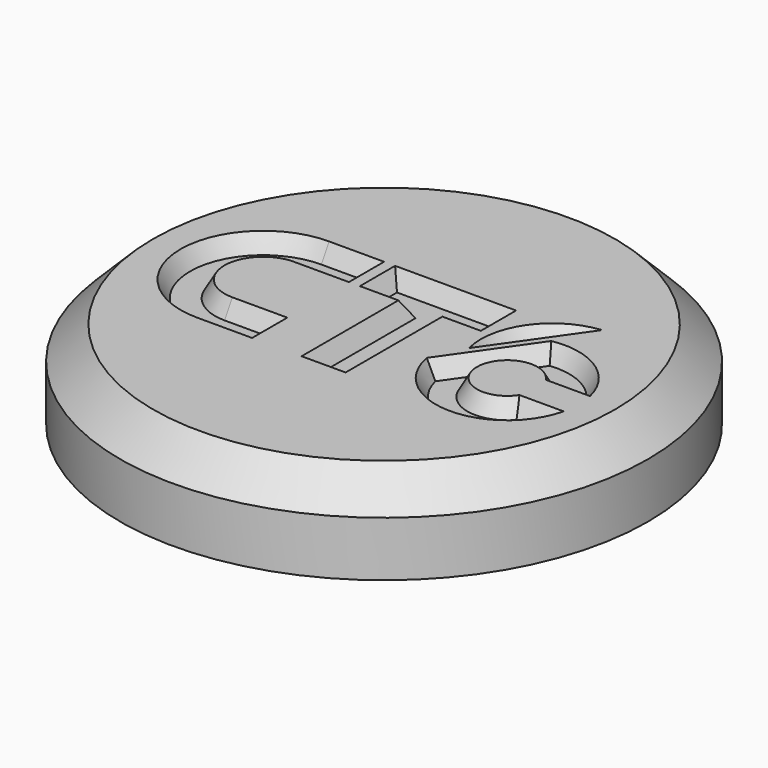
from build123d import *

# Parameters (mm, degrees)
F0_R                     = 24
F1_DEPTH                 = 8
F2_R                     = 21
F3_DEPTH                 = 5.1
F4_SIZE                  = 3
F6_DEPTH                 = 1.5
DRAFT_F6_DRAFTED_ANGLE   = 30
DRAFT_F6_2_DRAFTED_ANGLE = 30
DRAFT_F6_3_DRAFTED_ANGLE = 30
DRAFT_F6_4_DRAFTED_ANGLE = 30


# Not quite as in the source:
# - an extrude with a draft is written as a straight extrude whose walls are then drafted


with BuildPart() as f1:
    # F0 (on Top) → F1 (new body)
    with BuildSketch(Plane.XY):
        Circle(F0_R)
    extrude(amount=F1_DEPTH)

    # F2 (on face) → F3 (cut)
    with BuildSketch(Plane(origin=(0, 0, 0), x_dir=(1, 0, 0), z_dir=(0, 0, -1))):
        Circle(F2_R)
    extrude(amount=-F3_DEPTH, mode=Mode.SUBTRACT)

    # F4
    f4_edges = [f1.edges().sort_by_distance(p)[0] for p in [
        (-24, 0, 8),
    ]]
    chamfer(f4_edges, length=F4_SIZE)


with BuildPart() as f6_drafted:
    # F5 (on face) → F6 (new body)
    with BuildSketch(Plane.XY.offset(8)):
        with BuildLine():
            Line((-6, 7.5), (-11, 7.5))
            ThreePointArc((-11, 7.5), (-18.5, 0), (-11, -7.5))
            Line((-11, -7.5), (-6, -7.5))
            Line((-6, -7.5), (-6, -3.5))
            Line((-6, -3.5), (-11, -3.5))
            ThreePointArc((-11, -3.5), (-14.5, 0), (-11, 3.5))
            Line((-11, 3.5), (-6, 3.5))
            Line((-6, 3.5), (-6, 7.5))
        make_face()
    extrude(amount=-F6_DEPTH)

    # draft_F6_drafted
    draft_f6_drafted_walls = [f6_drafted.faces().sort_by_distance(p)[0] for p in [
        (-8.5, 3.5, 7),
        (-6, 5.5, 7),
        (-8.5, 7.5, 7),
        (-18.5, 0, 7),
        (-8.5, -7.5, 7),
        (-6, -5.5, 7),
        (-8.5, -3.5, 7),
        (-14.5, 0, 7),
    ]]
    draft(draft_f6_drafted_walls, neutral_plane=Plane(origin=(0, 0, 8), x_dir=(1, 0, 0), z_dir=(0, 0, -1)), angle=DRAFT_F6_DRAFTED_ANGLE)


with BuildPart() as f1_1:
    add(f1.part)

    # join_F6_drafted: cut F6_drafted
    add(f6_drafted.part, mode=Mode.SUBTRACT)


with BuildPart() as f6_2_drafted:
    # F5 (on face) → F6, piece 2 (new body)
    with BuildSketch(Plane.XY.offset(8)):
        Polygon((6, 7.5), (0.5, 7.5), (-5, 7.5), (-5, 3.5), (-1.5, 3.5), (-1.5, -7.5), (0.5, -7.5), (2.5, -7.5), (2.5, 3.5), (6, 3.5), align=None)
    extrude(amount=-F6_DEPTH)

    # draft_F6_2_drafted
    draft_f6_2_drafted_walls = [f6_2_drafted.faces().sort_by_distance(p)[0] for p in [
        (0.5, 7.5, 7),
        (4.25, 3.5, 7),
        (2.5, -2, 7),
        (0.5, -7.5, 7),
        (-1.5, -2, 7),
        (-3.25, 3.5, 7),
        (-5, 5.5, 7),
        (6, 5.5, 7),
    ]]
    draft(draft_f6_2_drafted_walls, neutral_plane=Plane(origin=(0, 0, 8), x_dir=(1, 0, 0), z_dir=(0, 0, -1)), angle=DRAFT_F6_2_DRAFTED_ANGLE)


with BuildPart() as f1_2:
    add(f1_1.part)

    # join_F6_2_drafted: cut F6_2_drafted
    add(f6_2_drafted.part, mode=Mode.SUBTRACT)


with BuildPart() as f6_3_drafted:
    # F5 (on face) → F6, piece 3 (new body)
    with BuildSketch(Plane.XY.offset(8)):
        with BuildLine():
            Line((14.3048861143, 0.5), (18.3245553203, 0.5))
            ThreePointArc((18.3245553203, 0.5), (15.575855344, 4.428006868), (10.8818401666, 5.4031022627))
            Line((10.8818401666, 5.4031022627), (5.6006188671, -2.1392634093))
            ThreePointArc((5.6006188671, -2.1392634093), (11.8157923793, -7.4973892874), (18.3245553203, -2.5))
            Line((18.3245553203, -2.5), (14.3048861143, -2.5))
            ThreePointArc((14.3048861143, -2.5), (9.25, -1), (14.3048861143, 0.5))
        make_face()
    extrude(amount=-F6_DEPTH)

    # draft_F6_3_drafted
    draft_f6_3_drafted_walls = [f6_3_drafted.faces().sort_by_distance(p)[0] for p in [
        (16.3147207173, -2.5, 7),
        (9.25, -1, 7),
        (16.3147207173, 0.5, 7),
        (15.575855344, 4.428006868, 7),
        (8.2412295169, 1.6319194267, 7),
        (11.8157923793, -7.4973892874, 7),
    ]]
    draft(draft_f6_3_drafted_walls, neutral_plane=Plane(origin=(0, 0, 8), x_dir=(1, 0, 0), z_dir=(0, 0, -1)), angle=DRAFT_F6_3_DRAFTED_ANGLE)


with BuildPart() as f1_3:
    add(f1_2.part)

    # join_F6_3_drafted: cut F6_3_drafted
    add(f6_3_drafted.part, mode=Mode.SUBTRACT)


with BuildPart() as f6_4_drafted:
    # F5 (on face) → F6, piece 4 (new body)
    with BuildSketch(Plane.XY.offset(8)):
        with BuildLine():
            Line((6.9990079566, 0.9039112589), (12.6447666104, 8.9668902268))
            ThreePointArc((12.6447666104, 8.9668902268), (7.9755117121, 6.2282468363), (6.9990079566, 0.9039112589))
        make_face()
    extrude(amount=-F6_DEPTH)

    # draft_F6_4_drafted
    draft_f6_4_drafted_walls = [f6_4_drafted.faces().sort_by_distance(p)[0] for p in [
        (7.9755117121, 6.2282468363, 7),
        (9.8218872835, 4.9354007428, 7),
    ]]
    draft(draft_f6_4_drafted_walls, neutral_plane=Plane(origin=(0, 0, 8), x_dir=(1, 0, 0), z_dir=(0, 0, -1)), angle=DRAFT_F6_4_DRAFTED_ANGLE)


with BuildPart() as f1_4:
    add(f1_3.part)

    # join_F6_4_drafted: cut F6_4_drafted
    add(f6_4_drafted.part, mode=Mode.SUBTRACT)


solid = f1_4.part
